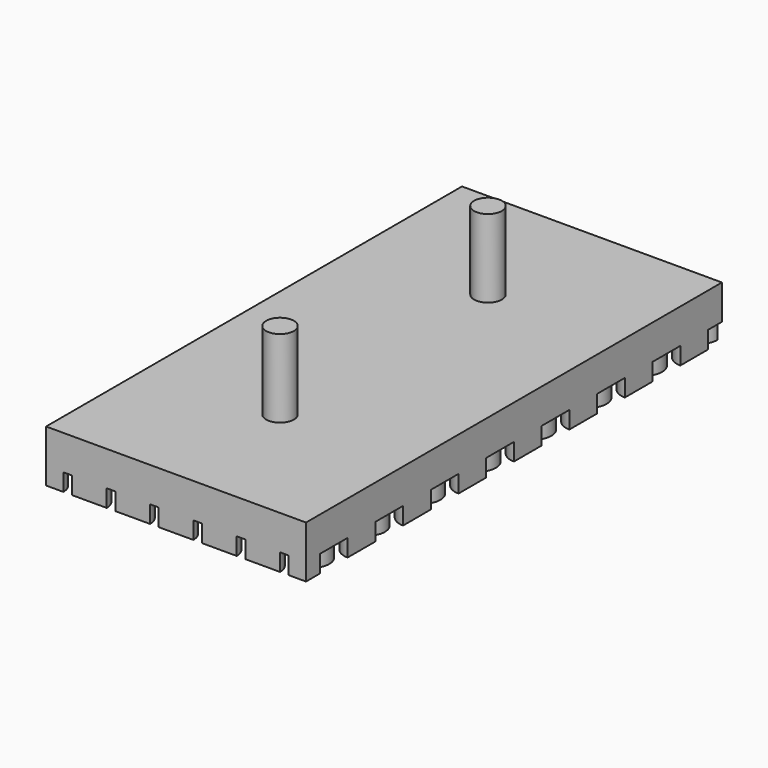
from build123d import *

# Parameters (mm, degrees)
F0_W     = 150
F0_H     = 300
F1_DEPTH = 20
F2_R     = 8
F3_DEPTH = 45
F4_R     = 10
F5_DEPTH = 10


with BuildPart() as f1:
    # F0 (on Top) → F1 (new body)
    with BuildSketch(Plane.XY):
        Rectangle(F0_W, F0_H)
    extrude(amount=-F1_DEPTH)

    # F2 (on face) → F3 (join)
    with BuildSketch(Plane.XY):
        with Locations((0, 75)):
            Circle(F2_R)
        with Locations((0, -75)):
            Circle(F2_R)
    extrude(amount=F3_DEPTH)

    # F4 (on face) → F5 (join)
    with BuildSketch(Plane(origin=(0, 0, -20), x_dir=(1, 0, 0), z_dir=(0, 0, -1))):
        with BuildLine():
            ThreePointArc((-75, 140.000005), (-67.9353975377, 142.9324686064), (-65.01, 150))
            Line((-65.01, 150), (-75, 150))
            Line((-75, 150), (-75, 140.000005))
        make_face()
        with BuildLine():
            Line((-40.01, 150), (-60.01, 150))
            ThreePointArc((-60.01, 150), (-50.01, 140), (-40.01, 150))
        make_face()
        with BuildLine():
            ThreePointArc((-65.01, 110), (-67.9353975377, 117.0675313936), (-75, 119.999995))
            Line((-75, 119.999995), (-75, 100.000005))
            ThreePointArc((-75, 100.000005), (-67.9353975377, 102.9324686064), (-65.01, 110))
        make_face()
        with BuildLine():
            Line((-15.01, 150), (-35.01, 150))
            ThreePointArc((-35.01, 150), (-25.01, 140), (-15.01, 150))
        make_face()
        with BuildLine():
            ThreePointArc((-65.01, 70), (-67.9353975377, 77.0675313936), (-75, 79.999995))
            Line((-75, 79.999995), (-75, 60.000005))
            ThreePointArc((-75, 60.000005), (-67.9353975377, 62.9324686064), (-65.01, 70))
        make_face()
        with BuildLine():
            Line((9.99, 150), (-10.01, 150))
            ThreePointArc((-10.01, 150), (-0.01, 140), (9.99, 150))
        make_face()
        with BuildLine():
            ThreePointArc((-65.01, 30), (-67.9353975377, 37.0675313936), (-75, 39.999995))
            Line((-75, 39.999995), (-75, 20.000005))
            ThreePointArc((-75, 20.000005), (-67.9353975377, 22.9324686064), (-65.01, 30))
        make_face()
        with BuildLine():
            Line((34.99, 150), (14.99, 150))
            ThreePointArc((14.99, 150), (24.99, 140), (34.99, 150))
        make_face()
        with BuildLine():
            ThreePointArc((-65.01, -10), (-67.9353975377, -2.9324686064), (-75, -5e-06))
            Line((-75, -5e-06), (-75, -19.999995))
            ThreePointArc((-75, -19.999995), (-67.9353975377, -17.0675313936), (-65.01, -10))
        make_face()
        with BuildLine():
            Line((59.99, 150), (39.99, 150))
            ThreePointArc((39.99, 150), (49.99, 140), (59.99, 150))
        make_face()
        with BuildLine():
            ThreePointArc((-65.01, -50), (-67.9353975377, -42.9324686064), (-75, -40.000005))
            Line((-75, -40.000005), (-75, -59.999995))
            ThreePointArc((-75, -59.999995), (-67.9353975377, -57.0675313936), (-65.01, -50))
        make_face()
        with BuildLine():
            Line((75, 150), (64.99, 150))
            ThreePointArc((64.99, 150), (67.9224686064, 142.9253975377), (75, 140.000005))
            Line((75, 140.000005), (75, 150))
        make_face()
        with BuildLine():
            ThreePointArc((-65.01, -90), (-67.9353975377, -82.9324686064), (-75, -80.000005))
            Line((-75, -80.000005), (-75, -99.999995))
            ThreePointArc((-75, -99.999995), (-67.9353975377, -97.0675313936), (-65.01, -90))
        make_face()
        with BuildLine():
            Line((75, 100.000005), (75, 119.999995))
            ThreePointArc((75, 119.999995), (64.99, 110), (75, 100.000005))
        make_face()
        with BuildLine():
            ThreePointArc((-65.01, -130), (-67.9353975377, -122.9324686064), (-75, -120.000005))
            Line((-75, -120.000005), (-75, -139.999995))
            ThreePointArc((-75, -139.999995), (-67.9353975377, -137.0675313936), (-65.01, -130))
        make_face()
        with BuildLine():
            Line((75, 60.000005), (75, 79.999995))
            ThreePointArc((75, 79.999995), (64.99, 70), (75, 60.000005))
        make_face()
        with BuildLine():
            ThreePointArc((-52.5, -150), (-62.5, -140), (-72.5, -150))
            Line((-72.5, -150), (-52.5, -150))
        make_face()
        with BuildLine():
            Line((75, 20.000005), (75, 39.999995))
            ThreePointArc((75, 39.999995), (64.99, 30), (75, 20.000005))
        make_face()
        with BuildLine():
            ThreePointArc((-27.5, -150), (-37.5, -140), (-47.5, -150))
            Line((-47.5, -150), (-27.5, -150))
        make_face()
        with BuildLine():
            Line((75, -19.999995), (75, -5e-06))
            ThreePointArc((75, -5e-06), (64.99, -10), (75, -19.999995))
        make_face()
        with BuildLine():
            ThreePointArc((-2.5, -150), (-12.5, -140), (-22.5, -150))
            Line((-22.5, -150), (-2.5, -150))
        make_face()
        with BuildLine():
            Line((75, -59.999995), (75, -40.000005))
            ThreePointArc((75, -40.000005), (64.99, -50), (75, -59.999995))
        make_face()
        with BuildLine():
            ThreePointArc((22.5, -150), (12.5, -140), (2.5, -150))
            Line((2.5, -150), (22.5, -150))
        make_face()
        with BuildLine():
            Line((75, -99.999995), (75, -80.000005))
            ThreePointArc((75, -80.000005), (64.99, -90), (75, -99.999995))
        make_face()
        with BuildLine():
            ThreePointArc((47.5, -150), (37.5, -140), (27.5, -150))
            Line((27.5, -150), (47.5, -150))
        make_face()
        with BuildLine():
            Line((75, -139.999995), (75, -120.000005))
            ThreePointArc((75, -120.000005), (64.99, -130), (75, -139.999995))
        make_face()
        with BuildLine():
            ThreePointArc((72.5, -150), (62.5, -140), (52.5, -150))
            Line((52.5, -150), (72.5, -150))
        make_face()
        with Locations((-62.5, 130)):
            Circle(F4_R)
        with Locations((-50.01, 110)):
            Circle(F4_R)
        with Locations((-50.01, 70)):
            Circle(F4_R)
        with Locations((-50.01, 30)):
            Circle(F4_R)
        with Locations((-50.01, -10)):
            Circle(F4_R)
        with Locations((-50.01, -50)):
            Circle(F4_R)
        with Locations((-50.01, -90)):
            Circle(F4_R)
        with Locations((-50.01, -130)):
            Circle(F4_R)
        with Locations((-25.01, 110)):
            Circle(F4_R)
        with Locations((-25.01, 70)):
            Circle(F4_R)
        with Locations((-25.01, 30)):
            Circle(F4_R)
        with Locations((-25.01, -10)):
            Circle(F4_R)
        with Locations((-25.01, -50)):
            Circle(F4_R)
        with Locations((-25.01, -90)):
            Circle(F4_R)
        with Locations((-25.01, -130)):
            Circle(F4_R)
        with Locations((-0.01, 110)):
            Circle(F4_R)
        with Locations((-0.01, 70)):
            Circle(F4_R)
        with Locations((-0.01, 30)):
            Circle(F4_R)
        with Locations((-0.01, -10)):
            Circle(F4_R)
        with Locations((-0.01, -50)):
            Circle(F4_R)
        with Locations((-0.01, -90)):
            Circle(F4_R)
        with Locations((-0.01, -130)):
            Circle(F4_R)
        with Locations((24.99, 110)):
            Circle(F4_R)
        with Locations((24.99, 70)):
            Circle(F4_R)
        with Locations((24.99, 30)):
            Circle(F4_R)
        with Locations((24.99, -10)):
            Circle(F4_R)
        with Locations((24.99, -50)):
            Circle(F4_R)
        with Locations((24.99, -90)):
            Circle(F4_R)
        with Locations((24.99, -130)):
            Circle(F4_R)
        with Locations((49.99, 110)):
            Circle(F4_R)
        with Locations((49.99, 70)):
            Circle(F4_R)
        with Locations((49.99, 30)):
            Circle(F4_R)
        with Locations((49.99, -10)):
            Circle(F4_R)
        with Locations((49.99, -50)):
            Circle(F4_R)
        with Locations((49.99, -90)):
            Circle(F4_R)
        with Locations((49.99, -130)):
            Circle(F4_R)
        with Locations((-62.5, 90)):
            Circle(F4_R)
        with Locations((-62.5, 50)):
            Circle(F4_R)
        with Locations((-62.5, 10)):
            Circle(F4_R)
        with Locations((-62.5, -30)):
            Circle(F4_R)
        with Locations((-62.5, -70)):
            Circle(F4_R)
        with Locations((-62.5, -110)):
            Circle(F4_R)
        with Locations((-37.5, 130)):
            Circle(F4_R)
        with Locations((-37.5, 90)):
            Circle(F4_R)
        with Locations((-37.5, 50)):
            Circle(F4_R)
        with Locations((-37.5, 10)):
            Circle(F4_R)
        with Locations((-37.5, -30)):
            Circle(F4_R)
        with Locations((-37.5, -70)):
            Circle(F4_R)
        with Locations((-37.5, -110)):
            Circle(F4_R)
        with Locations((-12.5, 130)):
            Circle(F4_R)
        with Locations((-12.5, 90)):
            Circle(F4_R)
        with Locations((-12.5, 50)):
            Circle(F4_R)
        with Locations((-12.5, 10)):
            Circle(F4_R)
        with Locations((-12.5, -30)):
            Circle(F4_R)
        with Locations((-12.5, -70)):
            Circle(F4_R)
        with Locations((-12.5, -110)):
            Circle(F4_R)
        with Locations((12.5, 130)):
            Circle(F4_R)
        with Locations((12.5, 90)):
            Circle(F4_R)
        with Locations((12.5, 50)):
            Circle(F4_R)
        with Locations((12.5, 10)):
            Circle(F4_R)
        with Locations((12.5, -30)):
            Circle(F4_R)
        with Locations((12.5, -70)):
            Circle(F4_R)
        with Locations((12.5, -110)):
            Circle(F4_R)
        with Locations((37.5, 130)):
            Circle(F4_R)
        with Locations((37.5, 90)):
            Circle(F4_R)
        with Locations((37.5, 50)):
            Circle(F4_R)
        with Locations((37.5, 10)):
            Circle(F4_R)
        with Locations((37.5, -30)):
            Circle(F4_R)
        with Locations((37.5, -70)):
            Circle(F4_R)
        with Locations((37.5, -110)):
            Circle(F4_R)
        with Locations((62.5, 130)):
            Circle(F4_R)
        with Locations((62.5, 90)):
            Circle(F4_R)
        with Locations((62.5, 50)):
            Circle(F4_R)
        with Locations((62.5, 10)):
            Circle(F4_R)
        with Locations((62.5, -30)):
            Circle(F4_R)
        with Locations((62.5, -70)):
            Circle(F4_R)
        with Locations((62.5, -110)):
            Circle(F4_R)
    extrude(amount=F5_DEPTH)


solid = f1.part
